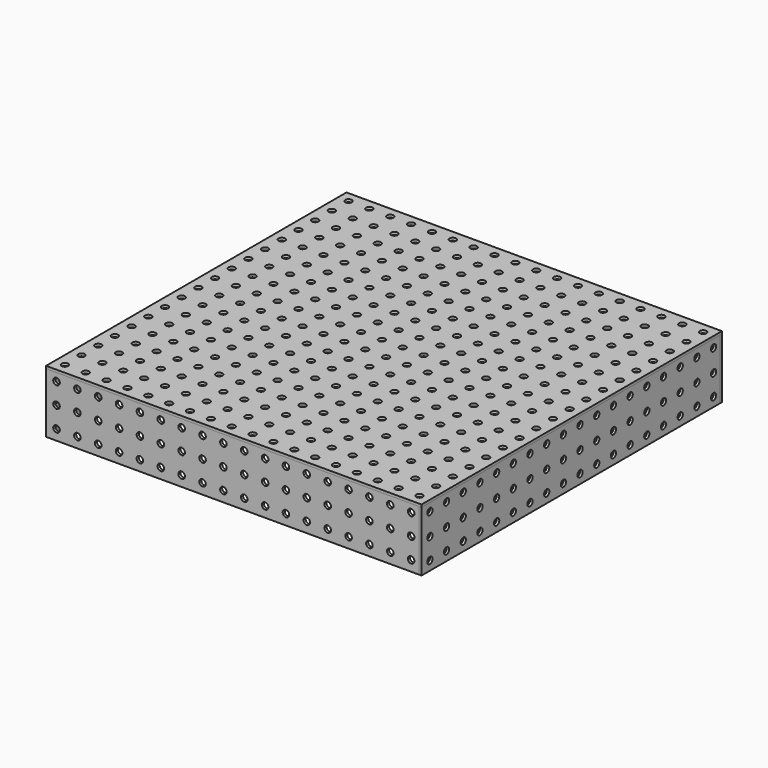
from build123d import *

# Parameters (mm, degrees)
F0_W      = 914.4
F0_H      = 914.4
F1_DEPTH  = 6.35
F3_D      = 16
F4_D      = 16
F5_D      = 16
F6_D      = 16
F7_D      = 16
F8_W      = 914.4
F8_H      = 146.05
F9_DEPTH  = 6.35
F10_W     = 914.4
F10_H     = 146.05
F11_DEPTH = 6.35
F12_W     = 914.4
F12_H     = 146.05
F13_DEPTH = 6.35
F14_W     = 914.4
F14_H     = 146.05
F15_DEPTH = 6.35
F18_D     = 16
F18_2_D   = 16
F20_D     = 16
F20_2_D   = 16


with BuildPart() as f1:
    # F0 (on Top) → F1 (new body)
    with BuildSketch(Plane.XY):
        Rectangle(F0_W, F0_H)
    extrude(amount=F1_DEPTH)

    # F3 (through all)
    with Locations(Plane.XY.offset(6.35)):
        with Locations((-431.8, 431.8), (-381, 431.8), (-330.2, 431.8), (-279.4, 431.8), (-228.6, 431.8), (-177.8, 431.8), (-127, 431.8), (-76.2, 431.8), (-25.4, 431.8), (25.4, 431.8), (76.2, 431.8), (127, 431.8), (177.8, 431.8), (228.6, 431.8), (279.4, 431.8), (330.2, 431.8), (381, 431.8), (431.8, 431.8), (431.8, 381), (381, 381), (330.2, 381), (279.4, 381), (228.6, 381), (177.8, 381), (127, 381), (76.2, 381), (25.4, 381), (-25.4, 381), (-76.2, 381), (-127, 381), (-177.8, 381), (-228.6, 381), (-279.4, 381), (-330.2, 381), (-381, 381), (-431.8, 381), (-431.8, 330.2), (-381, 330.2), (-330.2, 330.2), (-279.4, 330.2), (-228.6, 330.2), (-177.8, 330.2), (-127, 330.2), (-76.2, 330.2), (-25.4, 330.2), (25.4, 330.2), (76.2, 330.2), (127, 330.2), (177.8, 330.2), (228.6, 330.2), (279.4, 330.2), (330.2, 330.2), (381, 330.2), (431.8, 330.2), (431.8, 279.4), (381, 279.4), (330.2, 279.4), (279.4, 279.4), (228.6, 279.4), (177.8, 279.4), (127, 279.4), (76.2, 279.4), (25.4, 279.4), (-25.4, 279.4), (-76.2, 279.4), (-127, 279.4), (-177.8, 279.4), (-228.6, 279.4), (-279.4, 279.4), (-330.2, 279.4), (-381, 279.4), (-431.8, 279.4)):
            Hole(F3_D / 2)

    # F4 (through all)
    with Locations(Plane.XY.offset(6.35)):
        with Locations((-431.8, 228.6), (-431.8, 177.8), (-431.8, 127), (-431.8, 76.2), (-381, 76.2), (-381, 127), (-381, 177.8), (-381, 228.6), (-330.2, 228.6), (-330.2, 177.8), (-330.2, 127), (-330.2, 76.2), (-279.4, 76.2), (-279.4, 127), (-279.4, 177.8), (-279.4, 228.6), (-228.6, 228.6), (-228.6, 177.8), (-228.6, 127), (-228.6, 76.2), (-177.8, 76.2), (-177.8, 127), (-177.8, 177.8), (-177.8, 228.6), (-127, 228.6), (-127, 177.8), (-127, 127), (-127, 76.2), (-76.2, 76.2), (-76.2, 127), (-76.2, 177.8), (-76.2, 228.6), (-25.4, 228.6), (-25.4, 177.8), (-25.4, 127), (-25.4, 76.2), (25.4, 76.2), (25.4, 127), (25.4, 177.8), (25.4, 228.6), (76.2, 228.6), (76.2, 177.8), (76.2, 127), (76.2, 76.2), (127, 76.2), (127, 127), (127, 177.8), (127, 228.6), (177.8, 228.6), (177.8, 177.8), (177.8, 127), (177.8, 76.2), (228.6, 76.2), (228.6, 127), (228.6, 177.8), (228.6, 228.6), (279.4, 228.6), (279.4, 177.8), (279.4, 127), (279.4, 76.2), (330.2, 76.2), (330.2, 127), (330.2, 177.8), (330.2, 228.6), (381, 228.6), (381, 177.8), (381, 127), (381, 76.2), (431.8, 76.2), (431.8, 127), (431.8, 177.8), (431.8, 228.6)):
            Hole(F4_D / 2)

    # F5 (through all)
    with Locations(Plane.XY.offset(6.35)):
        with Locations((-431.8, 25.4), (-431.8, -25.4), (-431.8, -76.2), (-431.8, -127), (-381, -127), (-381, -76.2), (-381, -25.4), (-381, 25.4), (-330.2, 25.4), (-330.2, -25.4), (-330.2, -76.2), (-330.2, -127), (-279.4, -127), (-279.4, -76.2), (-279.4, -25.4), (-279.4, 25.4), (-228.6, 25.4), (-228.6, -25.4), (-228.6, -76.2), (-228.6, -127), (-177.8, -127), (-177.8, -76.2), (-177.8, -25.4), (-177.8, 25.4), (-127, 25.4), (-127, -25.4), (-127, -76.2), (-127, -127), (-76.2, -127), (-76.2, -76.2), (-76.2, -25.4), (-76.2, 25.4), (-25.4, 25.4), (-25.4, -25.4), (-25.4, -76.2), (-25.4, -127), (25.4, -127), (25.4, -76.2), (25.4, -25.4), (25.4, 25.4), (76.2, 25.4), (76.2, -25.4), (76.2, -76.2), (76.2, -127), (127, -127), (127, -76.2), (127, -25.4), (127, 25.4), (177.8, 25.4), (177.8, -25.4), (177.8, -76.2), (177.8, -127), (228.6, -127), (228.6, -76.2), (228.6, -25.4), (228.6, 25.4), (279.4, 25.4), (279.4, -25.4), (279.4, -76.2), (279.4, -127), (330.2, -127), (330.2, -76.2), (330.2, -25.4), (330.2, 25.4), (381, 25.4), (381, -25.4), (381, -76.2), (381, -127), (431.8, -127), (431.8, -76.2), (431.8, -25.4), (431.8, 25.4)):
            Hole(F5_D / 2)

    # F6 (through all)
    with Locations(Plane.XY.offset(6.35)):
        with Locations((-431.8, -177.8), (-431.8, -228.6), (-431.8, -279.4), (-431.8, -330.2), (-381, -177.8), (-381, -228.6), (-381, -279.4), (-381, -330.2), (-330.2, -177.8), (-330.2, -228.6), (-330.2, -279.4), (-330.2, -330.2), (-279.4, -330.2), (-279.4, -279.4), (-279.4, -228.6), (-279.4, -177.8), (-228.6, -177.8), (-228.6, -228.6), (-228.6, -279.4), (-228.6, -330.2), (-177.8, -330.2), (-177.8, -279.4), (-177.8, -228.6), (-177.8, -177.8), (-127, -177.8), (-127, -228.6), (-127, -279.4), (-127, -330.2), (-76.2, -330.2), (-76.2, -279.4), (-76.2, -228.6), (-76.2, -177.8), (-25.4, -177.8), (-25.4, -228.6), (-25.4, -279.4), (-25.4, -330.2), (25.4, -330.2), (25.4, -279.4), (25.4, -228.6), (25.4, -177.8), (76.2, -177.8), (76.2, -228.6), (76.2, -279.4), (76.2, -330.2), (127, -330.2), (127, -279.4), (127, -228.6), (127, -177.8), (177.8, -177.8), (177.8, -228.6), (177.8, -330.2), (177.8, -279.4), (228.6, -330.2), (228.6, -279.4), (228.6, -228.6), (228.6, -177.8), (279.4, -177.8), (279.4, -228.6), (279.4, -279.4), (279.4, -330.2), (330.2, -330.2), (381, -279.4), (431.8, -228.6), (381, -177.8), (330.2, -228.6), (431.8, -330.2), (381, -330.2), (431.8, -279.4), (381, -228.6), (330.2, -177.8), (431.8, -177.8), (330.2, -279.4)):
            Hole(F6_D / 2)

    # F7 (through all)
    with Locations(Plane.XY.offset(6.35)):
        with Locations((-431.8, -381), (-381, -381), (-330.2, -381), (-279.4, -381), (-228.6, -381), (-177.8, -381), (-127, -381), (-76.2, -381), (-25.4, -381), (25.4, -381), (76.2, -381), (127, -381), (177.8, -381), (228.6, -381), (279.4, -381), (330.2, -381), (381, -381), (431.8, -381), (-431.8, -431.8), (-381, -431.8), (-330.2, -431.8), (-279.4, -431.8), (-228.6, -431.8), (-177.8, -431.8), (-127, -431.8), (-76.2, -431.8), (-25.4, -431.8), (25.4, -431.8), (76.2, -431.8), (127, -431.8), (177.8, -431.8), (228.6, -431.8), (279.4, -431.8), (330.2, -431.8), (381, -431.8), (431.8, -431.8)):
            Hole(F7_D / 2)


with BuildPart() as f9:
    # F8 (on face) → F9 (new body)
    with BuildSketch(Plane(origin=(-457.2, 0, 0), x_dir=(0, -1, 0), z_dir=(-1, 0, 0))):
        with Locations((0, -73.025)):
            Rectangle(F8_W, F8_H)
    extrude(amount=-F9_DEPTH)

    # F10 (on face) → F11 (join)
    with BuildSketch(Plane.XZ.offset(457.2)):
        with Locations((0, -73.025)):
            Rectangle(F10_W, F10_H)
    extrude(amount=-F11_DEPTH)

    # F18 (through all)
    with Locations(Plane(origin=(-457.2, 0, 0), x_dir=(0, -1, 0), z_dir=(-1, 0, 0))):
        with Locations((-431.8, -19.05), (-381, -19.05), (-330.2, -19.05), (-279.4, -19.05), (-228.6, -19.05), (-177.8, -19.05), (-127, -19.05), (-76.2, -19.05), (-25.4, -19.05), (25.4, -19.05), (76.2, -19.05), (127, -19.05), (177.8, -19.05), (228.6, -19.05), (279.4, -19.05), (330.2, -19.05), (381, -19.05), (431.8, -19.05), (-431.8, -73.025), (-381, -73.025), (-330.2, -73.025), (-279.4, -73.025), (-228.6, -73.025), (-177.8, -73.025), (-127, -73.025), (-76.2, -73.025), (-25.4, -73.025), (25.4, -73.025), (76.2, -73.025), (127, -73.025), (177.8, -73.025), (228.6, -73.025), (279.4, -73.025), (330.2, -73.025), (381, -73.025), (431.8, -73.025), (-431.8, -123.825), (-381, -123.825), (-330.2, -123.825), (-279.4, -123.825), (-228.6, -123.825), (-177.8, -123.825), (-127, -123.825), (-76.2, -123.825), (-25.4, -123.825), (25.4, -123.825), (76.2, -123.825), (127, -123.825), (177.8, -123.825), (228.6, -123.825), (279.4, -123.825), (330.2, -123.825), (381, -123.825), (431.8, -123.825)):
            Hole(F18_D / 2)

    # F20 (through all)
    with Locations(Plane.XZ.offset(457.2)):
        with Locations((-431.8, -19.05), (-381, -19.05), (-330.2, -19.05), (-279.4, -19.05), (-228.6, -19.05), (-177.8, -19.05), (-127, -19.05), (-76.2, -19.05), (-25.4, -19.05), (25.4, -19.05), (76.2, -19.05), (127, -19.05), (177.8, -19.05), (228.6, -19.05), (279.4, -19.05), (330.2, -19.05), (381, -19.05), (431.8, -19.05), (-431.8, -69.85), (-381, -68.698388309), (-330.2, -69.85), (-279.4, -69.85), (-228.6, -69.85), (-177.8, -69.85), (-127, -69.85), (-76.2, -69.85), (-25.4, -69.85), (25.4, -69.85), (76.2, -69.85), (127, -69.85), (177.8, -69.85), (228.6, -69.85), (279.4, -69.85), (330.2, -69.85), (381, -69.85), (431.8, -69.85), (431.8, -120.65), (381, -120.65), (330.2, -120.65), (279.4, -120.65), (228.6, -120.65), (177.8, -120.65), (127, -120.65), (76.2, -120.65), (25.4, -120.65), (-25.4, -120.65), (-76.2, -120.65), (-127, -120.65), (-177.8, -120.65), (-228.6, -120.65), (-279.4, -120.65), (-330.2, -120.65), (-381, -120.65), (-431.8, -120.65)):
            Hole(F20_D / 2)


with BuildPart() as f13:
    # F12 (on face) → F13 (new body)
    with BuildSketch(Plane.YZ.offset(457.2)):
        with Locations((0, -73.025)):
            Rectangle(F12_W, F12_H)
    extrude(amount=-F13_DEPTH)

    # F18#2 (through all)
    with Locations(Plane(origin=(-457.2, 0, 0), x_dir=(0, -1, 0), z_dir=(-1, 0, 0))):
        with Locations((-431.8, -19.05), (-381, -19.05), (-330.2, -19.05), (-279.4, -19.05), (-228.6, -19.05), (-177.8, -19.05), (-127, -19.05), (-76.2, -19.05), (-25.4, -19.05), (25.4, -19.05), (76.2, -19.05), (127, -19.05), (177.8, -19.05), (228.6, -19.05), (279.4, -19.05), (330.2, -19.05), (381, -19.05), (431.8, -19.05), (-431.8, -73.025), (-381, -73.025), (-330.2, -73.025), (-279.4, -73.025), (-228.6, -73.025), (-177.8, -73.025), (-127, -73.025), (-76.2, -73.025), (-25.4, -73.025), (25.4, -73.025), (76.2, -73.025), (127, -73.025), (177.8, -73.025), (228.6, -73.025), (279.4, -73.025), (330.2, -73.025), (381, -73.025), (431.8, -73.025), (-431.8, -123.825), (-381, -123.825), (-330.2, -123.825), (-279.4, -123.825), (-228.6, -123.825), (-177.8, -123.825), (-127, -123.825), (-76.2, -123.825), (-25.4, -123.825), (25.4, -123.825), (76.2, -123.825), (127, -123.825), (177.8, -123.825), (228.6, -123.825), (279.4, -123.825), (330.2, -123.825), (381, -123.825), (431.8, -123.825)):
            Hole(F18_2_D / 2)


with BuildPart() as f15:
    # F14 (on face) → F15 (new body)
    with BuildSketch(Plane(origin=(0, 457.2, 0), x_dir=(-1, 0, 0), z_dir=(0, 1, 0))):
        with Locations((0, -73.025)):
            Rectangle(F14_W, F14_H)
    extrude(amount=-F15_DEPTH)

    # F20#2 (through all)
    with Locations(Plane.XZ.offset(457.2)):
        with Locations((-431.8, -19.05), (-381, -19.05), (-330.2, -19.05), (-279.4, -19.05), (-228.6, -19.05), (-177.8, -19.05), (-127, -19.05), (-76.2, -19.05), (-25.4, -19.05), (25.4, -19.05), (76.2, -19.05), (127, -19.05), (177.8, -19.05), (228.6, -19.05), (279.4, -19.05), (330.2, -19.05), (381, -19.05), (431.8, -19.05), (-431.8, -69.85), (-381, -68.698388309), (-330.2, -69.85), (-279.4, -69.85), (-228.6, -69.85), (-177.8, -69.85), (-127, -69.85), (-76.2, -69.85), (-25.4, -69.85), (25.4, -69.85), (76.2, -69.85), (127, -69.85), (177.8, -69.85), (228.6, -69.85), (279.4, -69.85), (330.2, -69.85), (381, -69.85), (431.8, -69.85), (431.8, -120.65), (381, -120.65), (330.2, -120.65), (279.4, -120.65), (228.6, -120.65), (177.8, -120.65), (127, -120.65), (76.2, -120.65), (25.4, -120.65), (-25.4, -120.65), (-76.2, -120.65), (-127, -120.65), (-177.8, -120.65), (-228.6, -120.65), (-279.4, -120.65), (-330.2, -120.65), (-381, -120.65), (-431.8, -120.65)):
            Hole(F20_2_D / 2)


solid = Compound([f1.part, f9.part, f13.part, f15.part])
